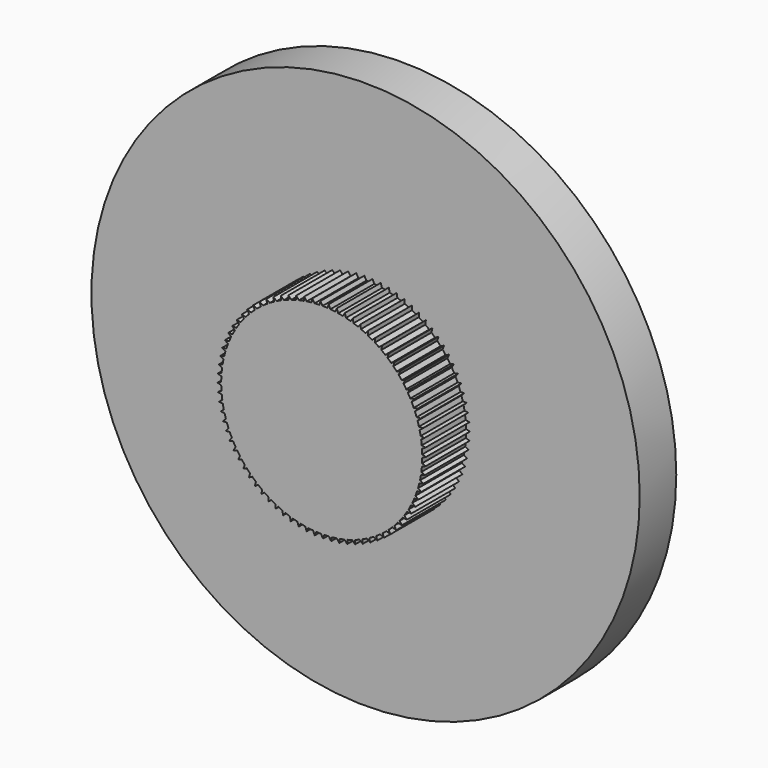
from build123d import *

# Parameters (mm, degrees)
F1_R            = 11
F2_DEPTH        = 11
F0_R            = 30
F3_DEPTH        = 5
F5_DEPTH        = 6.29
F5_COPIES_COUNT = 80


# Not quite as in the source:
# - a pattern or mirror of a feature is missing from the dataset's text; its kind, count and spacing are read off the source's solid


with BuildPart() as f2:
    # F1 (on Front) → F2 (new body)
    with BuildSketch(Plane.XZ):
        Circle(F1_R)
    extrude(amount=F2_DEPTH)

    # F0 (on Front) → F3 (join)
    with BuildSketch(Plane.XZ):
        Circle(F0_R)
    extrude(amount=F3_DEPTH)

    # F4 (on face) → F5 (join)
    with BuildSketch(Plane.XZ.offset(11)):
        with BuildLine():
            Line((-11.1250480992, 2.5344335095), (-10.7502806533, 2.3305505519))
            ThreePointArc((-10.7502806533, 2.3305505519), (-10.7146459859, 2.4892491631), (-10.6766687004, 2.6474035322))
            Line((-10.6766687004, 2.6474035322), (-11.1250480992, 2.5344335095))
        make_face()
    f5 = extrude(amount=-F5_DEPTH)

    # F5_copies: F5 ×80 about axis
    f5_copies_axis = Axis((0, 0, 0), (0, 1, 0))
    for i in range(1, F5_COPIES_COUNT):
        add(f5.rotate(f5_copies_axis, i * 360 / F5_COPIES_COUNT))


solid = f2.part
